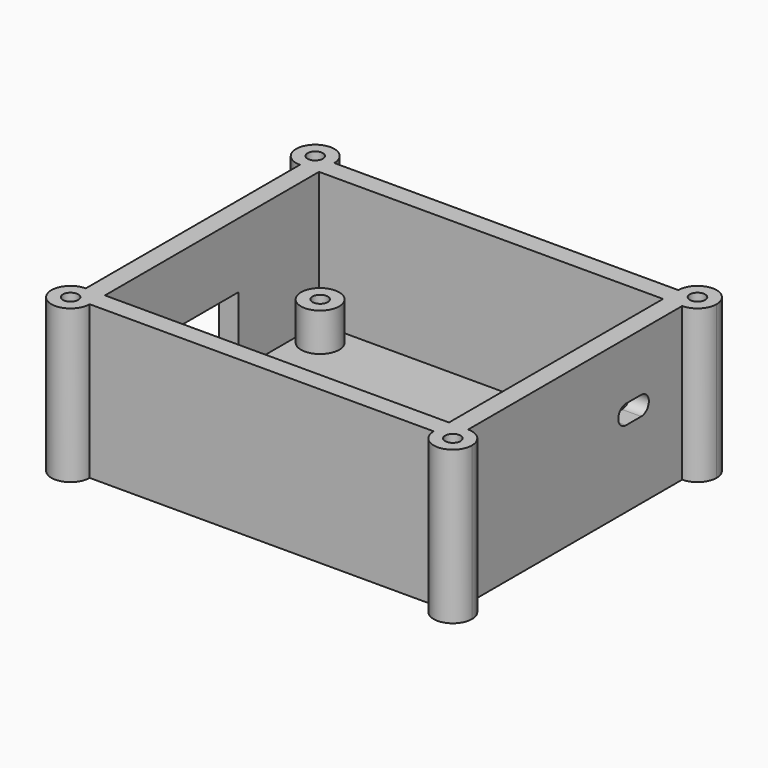
from build123d import *

# Parameters (mm, degrees)
F1_DEPTH        = 20
F2_T            = 2.5
F2_T3_DEPTH     = 25
F3_R            = 2.5
F4_DEPTH        = 5
F11_W           = 3
F11_H           = 2
F12_DEPTH       = 5
F13_DEPTH       = 5
F14_W           = 11
F14_H           = 9
F15_DEPTH       = 5
F16_D           = 2
F16_DEPTH       = 10
F16_TIP         = 0.600860619
F17_D           = 2
F17_DEPTH       = 5
F17_TIP         = 0.600860619
F17_ON_F7_D     = 2
F17_ON_F7_DEPTH = 5
F17_ON_F7_TIP   = 0.600860619
F17_ON_F6_D     = 2
F17_ON_F6_DEPTH = 5
F17_ON_F6_TIP   = 0.600860619
F17_ON_F8_D     = 2
F17_ON_F8_DEPTH = 5
F17_ON_F8_TIP   = 0.600860619


# Not quite as in the source:
# - a shell that OpenCascade refuses in one call is made with other operations: the cavity is built on its own and cut out


with BuildPart() as f1:
    # F0 (on Top) → F1 (new body)
    with BuildSketch(Plane.XY):
        with BuildLine():
            Line((-25, 17.5), (-25, 20))
            Line((-25, 20), (-22.5, 20))
            ThreePointArc((-22.5, 20), (-26.767766953, 21.767766953), (-25, 17.5))
        make_face()
        with BuildLine():
            Line((-22.5, 20), (-25, 20))
            Line((-25, 20), (-25, 17.5))
            ThreePointArc((-25, 17.5), (-23.232233047, 18.232233047), (-22.5, 20))
        make_face()
        with BuildLine():
            Line((22.5, 20), (-22.5, 20))
            ThreePointArc((-22.5, 20), (-23.232233047, 18.232233047), (-25, 17.5))
            Line((-25, 17.5), (-25, -17.5))
            ThreePointArc((-25, -17.5), (-23.232233047, -18.232233047), (-22.5, -20))
            Line((-22.5, -20), (22.5, -20))
            ThreePointArc((22.5, -20), (23.232233047, -18.232233047), (25, -17.5))
            Line((25, -17.5), (25, 17.5))
            ThreePointArc((25, 17.5), (23.232233047, 18.232233047), (22.5, 20))
        make_face()
        with BuildLine():
            ThreePointArc((27.5, 20), (25, 22.5), (22.5, 20))
            Line((22.5, 20), (25, 20))
            Line((25, 20), (25, 17.5))
            ThreePointArc((25, 17.5), (26.767766953, 18.232233047), (27.5, 20))
        make_face()
        with BuildLine():
            Line((25, 20), (22.5, 20))
            ThreePointArc((22.5, 20), (23.232233047, 18.232233047), (25, 17.5))
            Line((25, 17.5), (25, 20))
        make_face()
        with BuildLine():
            ThreePointArc((-22.5, -20), (-23.232233047, -18.232233047), (-25, -17.5))
            Line((-25, -17.5), (-25, -20))
            Line((-25, -20), (-22.5, -20))
        make_face()
        with BuildLine():
            Line((-25, -20), (-25, -17.5))
            ThreePointArc((-25, -17.5), (-26.767766953, -21.767766953), (-22.5, -20))
            Line((-22.5, -20), (-25, -20))
        make_face()
        with BuildLine():
            ThreePointArc((27.5, -20), (26.767766953, -18.232233047), (25, -17.5))
            Line((25, -17.5), (25, -20))
            Line((25, -20), (22.5, -20))
            ThreePointArc((22.5, -20), (25, -22.5), (27.5, -20))
        make_face()
        with BuildLine():
            Line((25, -20), (25, -17.5))
            ThreePointArc((25, -17.5), (23.232233047, -18.232233047), (22.5, -20))
            Line((22.5, -20), (25, -20))
        make_face()
    extrude(amount=F1_DEPTH)

    # F2: shell of thickness 2.5, made by hand


with BuildPart() as f2_core1:
    # F2_t2: copy of F1
    add(f1.part)

    # the walls: a layer under each face that stays
    f2_faces = [f2_core1.faces().sort_by_distance(p)[0] for p in [
        (-25, 0, 10),
        (0, -20, 10),
        (25, 0, 10),
        (0, 20, 10),
        (0, 0, 0),
    ]]
    thicken(f2_faces, amount=-F2_T, mode=Mode.SUBTRACT)

    # F2_s4 → F2_t3 (cut)
    with BuildSketch(Plane.XY.offset(-2.5)):
        Polygon((-22.475, 20.025), (-25, 20), (-25, 17.5), (-22.5, 17.5), align=None)
        Polygon((-25.025, 17.475), (-25, 20), (-22.5, 20), (-22.5, 17.5), align=None)
        Polygon((-25.025, -17.475), (-22.5, -17.5), (-22.5, -20), (-25, -20), align=None)
        Polygon((-22.475, -20.025), (-25, -20), (-25, -17.5), (-22.5, -17.5), align=None)
        Polygon((22.475, -20.025), (22.5, -17.5), (25, -17.5), (25, -20), align=None)
        Polygon((25.025, -17.475), (25, -20), (22.5, -20), (22.5, -17.5), align=None)
        Polygon((25.025, 17.475), (22.5, 17.5), (22.5, 20), (25, 20), align=None)
        Polygon((22.475, 20.025), (25, 20), (25, 17.5), (22.5, 17.5), align=None)
    extrude(amount=F2_T3_DEPTH, mode=Mode.SUBTRACT)


with BuildPart() as f1_1:
    add(f1.part)

    # what is left inside the walls is the cavity
    f2_cavity = [f2_core1.part.solids().sort_by_distance(p)[0] for p in [
        (0, -5.833333, 2.525),
    ]]
    add(f2_cavity, mode=Mode.SUBTRACT)

    # F3 (on face) → F4 (join)
    with BuildSketch(Plane.XY.offset(2.5)):
        with Locations((-19.8, 14.3)):
            Circle(F3_R)
        with Locations((19.8, 14.3)):
            Circle(F3_R)
        with Locations((-19.8, -14.3)):
            Circle(F3_R)
        with Locations((19.8, -14.3)):
            Circle(F3_R)
    extrude(amount=F4_DEPTH)

    # F11 (on face) → F12 (cut)
    with BuildSketch(Plane(origin=(0, 20, 0), x_dir=(-1, 0, 0), z_dir=(0, 1, 0))):
        with Locations((-7.3, 4.5)):
            Rectangle(F11_W, F11_H)
    extrude(amount=-F12_DEPTH, mode=Mode.SUBTRACT)

    # F10 (on face) → F13 (cut)
    with BuildSketch(Plane.YZ.offset(25)):
        with BuildLine():
            Line((10.8, 12.5), (8.3, 12.5))
            ThreePointArc((8.3, 12.5), (7.05, 11.25), (8.3, 10))
            Line((8.3, 10), (10.8, 10))
            ThreePointArc((10.8, 10), (12.05, 11.25), (10.8, 12.5))
        make_face()
    extrude(amount=-F13_DEPTH, mode=Mode.SUBTRACT)

    # F14 (on face) → F15 (cut)
    with BuildSketch(Plane(origin=(-25, 0, 0), x_dir=(0, -1, 0), z_dir=(-1, 0, 0))):
        with Locations((1.2, 7)):
            Rectangle(F14_W, F14_H)
    extrude(amount=-F15_DEPTH, mode=Mode.SUBTRACT)

    # F16
    with Locations(Plane.XY.offset(20)):
        with Locations((-25, 20), (25, 20), (-25, -20), (25, -20)):
            Hole(F16_D / 2, depth=F16_DEPTH)
            with Locations((0, 0, -(F16_DEPTH + F16_TIP / 2))):  # 118° drill point
                Cone(0, F16_D / 2, F16_TIP, mode=Mode.SUBTRACT)

    # F17
    with Locations(Plane.XY.offset(7.5)):
        with Locations((-19.8, 14.3)):
            Hole(F17_D / 2, depth=F17_DEPTH)
            with Locations((0, 0, -(F17_DEPTH + F17_TIP / 2))):  # 118° drill point
                Cone(0, F17_D / 2, F17_TIP, mode=Mode.SUBTRACT)

    # F17 on F7
    with Locations(Plane.XY.offset(7.5)):
        with Locations((19.8, 14.3)):
            Hole(F17_ON_F7_D / 2, depth=F17_ON_F7_DEPTH)
            with Locations((0, 0, -(F17_ON_F7_DEPTH + F17_ON_F7_TIP / 2))):  # 118° drill point
                Cone(0, F17_ON_F7_D / 2, F17_ON_F7_TIP, mode=Mode.SUBTRACT)

    # F17 on F6
    with Locations(Plane.XY.offset(7.5)):
        with Locations((-19.8, -14.3)):
            Hole(F17_ON_F6_D / 2, depth=F17_ON_F6_DEPTH)
            with Locations((0, 0, -(F17_ON_F6_DEPTH + F17_ON_F6_TIP / 2))):  # 118° drill point
                Cone(0, F17_ON_F6_D / 2, F17_ON_F6_TIP, mode=Mode.SUBTRACT)

    # F17 on F8
    with Locations(Plane.XY.offset(7.5)):
        with Locations((19.8, -14.3)):
            Hole(F17_ON_F8_D / 2, depth=F17_ON_F8_DEPTH)
            with Locations((0, 0, -(F17_ON_F8_DEPTH + F17_ON_F8_TIP / 2))):  # 118° drill point
                Cone(0, F17_ON_F8_D / 2, F17_ON_F8_TIP, mode=Mode.SUBTRACT)


solid = f1_1.part
